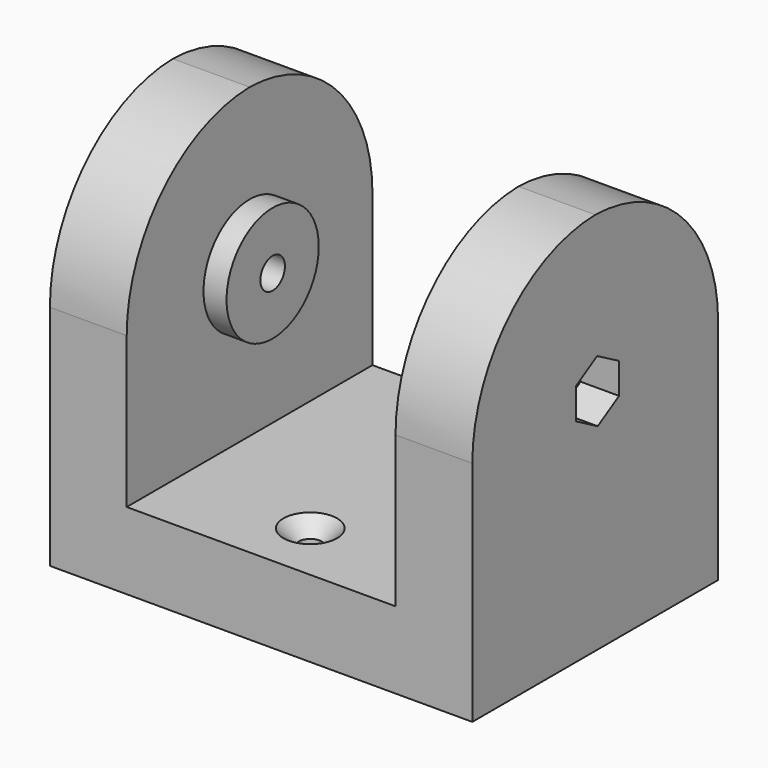
from build123d import *

# Parameters (mm, degrees)
F0_W           = 55
F0_H           = 40
F12_DEPTH      = 50
F1_W           = 35
F1_H           = 40
F13_DEPTH      = 40.001
F14_T1_DEPTH   = 111.7855168217
F14_T3_DEPTH   = 111.7855168217
F15_R          = 2
F2_DEPTH       = 55.001
F3_R           = 7.5
F3_R_2         = 2
F16_DEPTH      = 3
F6_D           = 3
F6_CSINK_D     = 7
F6_CSINK_ANGLE = 90
F7_R           = 2
F8_DEPTH       = 5
F17_R          = 4
F17_R_2        = 2
F9_DEPTH       = 5


# Not quite as in the source:
# - a fillet or chamfer that OpenCascade refuses, or shapes differently, is made with other operations: its cross-section is extruded or revolved along the edge and cut away or added


with BuildPart() as f12:
    # F0 (on Top) → F12 (new body)
    with BuildSketch(Plane.XY):
        Rectangle(F0_W, F0_H)
    extrude(amount=F12_DEPTH)

    # F1 (on face) → F13 (cut, through all)
    with BuildSketch(Plane.XZ.offset(20)):
        with Locations((0, 30)):
            Rectangle(F1_W, F1_H)
    extrude(amount=-F13_DEPTH, mode=Mode.SUBTRACT)

    # F14: fillet of radius 20.3571033643 on 4 edges, made by hand

    # F14_s2 → F14_t1 (cut)
    with BuildSketch(Plane.YZ.offset(-33.3927584109)):
        with BuildLine():
            ThreePointArc((-20, 29.6428966357), (-14.0375424699, 44.0375424699), (0.3571033643, 50))
            Line((0.3571033643, 50), (-20, 50))
            Line((-20, 50), (-20, 29.6428966357))
        make_face()
        with BuildLine():
            ThreePointArc((-0.3571033643, 50), (14.0375424699, 44.0375424699), (20, 29.6428966357))
            Line((20, 29.6428966357), (20, 50))
            Line((20, 50), (-0.3571033643, 50))
        make_face()
    extrude(amount=F14_T1_DEPTH, mode=Mode.SUBTRACT)

    # F14_s4 → F14_t3 (cut)
    with BuildSketch(Plane.YZ.offset(-78.3927584109)):
        with BuildLine():
            ThreePointArc((-20, 29.6428966357), (-14.0375424699, 44.0375424699), (0.3571033643, 50))
            Line((0.3571033643, 50), (-20, 50))
            Line((-20, 50), (-20, 29.6428966357))
        make_face()
        with BuildLine():
            ThreePointArc((-0.3571033643, 50), (14.0375424699, 44.0375424699), (20, 29.6428966357))
            Line((20, 29.6428966357), (20, 50))
            Line((20, 50), (-0.3571033643, 50))
        make_face()
    extrude(amount=F14_T3_DEPTH, mode=Mode.SUBTRACT)

    # F15 (on face) → F2 (cut, through all)
    with BuildSketch(Plane.YZ.offset(27.5)):
        with Locations((0, 29.6428966357)):
            Circle(F15_R)
    extrude(amount=-F2_DEPTH, mode=Mode.SUBTRACT)

    # F3 (on face) → F16 (join)
    with BuildSketch(Plane.YZ.offset(-17.5)):
        with Locations((0, 29.6428966357)):
            Circle(F3_R)
        with Locations((0, 29.6428966357)):
            Circle(F3_R_2, mode=Mode.SUBTRACT)
    extrude(amount=F16_DEPTH)

    # F4: F12 across plane


with BuildPart() as f12_1:
    add(f12.part)
    add(f12.part.mirror(Plane.YZ))

    # F6 (through all)
    with Locations(Plane.XY.offset(10)):
        with Locations((0, 12), (0, -12)):
            CounterSinkHole(F6_D / 2, F6_CSINK_D / 2, counter_sink_angle=F6_CSINK_ANGLE)

    # F7 (on face) → F8 (cut)
    with BuildSketch(Plane.YZ.offset(27.5)):
        Polygon((0.4025775089, 25.6017005954), (3.8796188691, 27.6616803799), (3.8341447246, 31.7028764202), (0.3116292198, 33.6840926759), (-3.1654121404, 31.6241128914), (-3.1199379959, 27.5829168512), align=None)
        with Locations((0, 29.6428966357)):
            Circle(F7_R, mode=Mode.SUBTRACT)
    extrude(amount=-F8_DEPTH, mode=Mode.SUBTRACT)

    # F17 (on face) → F9 (cut)
    with BuildSketch(Plane(origin=(-27.5, 0, 0), x_dir=(0, -1, 0), z_dir=(-1, 0, 0))):
        with Locations((0, 29.6428966357)):
            Circle(F17_R)
        with Locations((0, 29.6428966357)):
            Circle(F17_R_2, mode=Mode.SUBTRACT)
    extrude(amount=-F9_DEPTH, mode=Mode.SUBTRACT)


solid = f12_1.part
